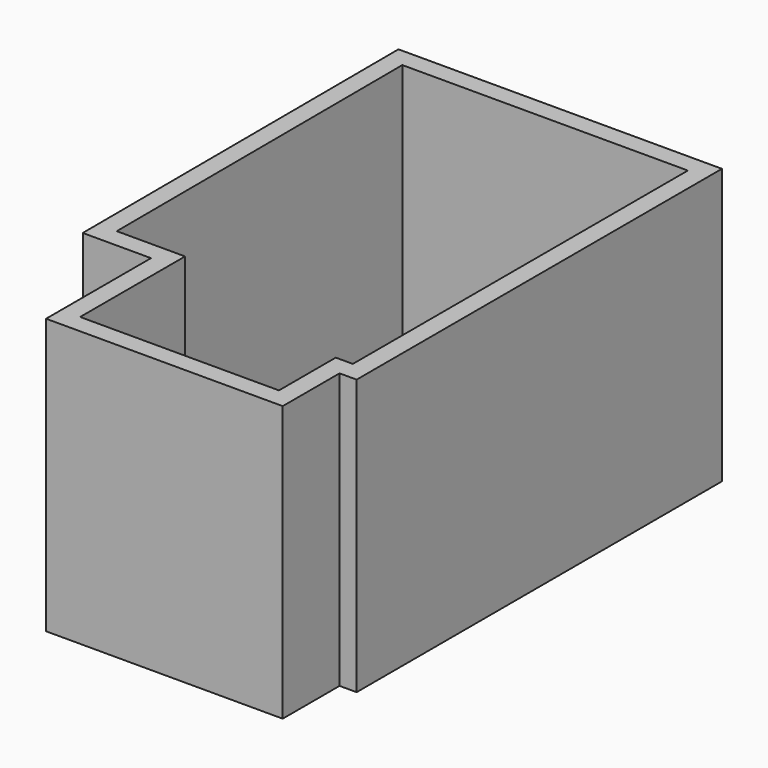
from build123d import *

# Parameters (mm, degrees)
F1_DEPTH = 25
F2_DEPTH = 2800
F3_W     = 800
F3_H     = 2000
F4_DEPTH = 199.3887424469
F5_DEPTH = 100


with BuildPart() as f1:
    # F0 (on Top) → F1 (new body)
    with BuildSketch(Plane.XY):
        Polygon((-1491.7285442352, 67.914776504), (-1477.3293733597, -3711.8628025055), (-757.3717832565, -3711.8628025055), (-757.3717832565, -5094.1815376282), (1337.7048969269, -5094.1815376282), (1337.7048969269, -4345.4256057739), (1517.6943540573, -4345.4256057739), (1517.6943540573, 67.914776504), align=None)
    extrude(amount=-F1_DEPTH)


with BuildPart() as f2:
    # F0 (on Top) → F2 (new body)
    with BuildSketch(Plane.XY):
        Polygon((1537.0936393738, -5293.5702800751), (1537.0936393738, -4544.8143482208), (1717.0830965042, -4544.8143482208), (1717.0830965042, 267.3035189509), (-1691.8783106137, 267.3035189509), (-1675.9599854953, -3911.2515449524), (-956.7605257034, -3911.2515449524), (-956.7605257034, -5293.5702800751), align=None)
        Polygon((-757.3717832565, -3711.8628025055), (-1477.3293733597, -3711.8628025055), (-1491.7285442352, 67.914776504), (1517.6943540573, 67.914776504), (1517.6943540573, -4345.4256057739), (1337.7048969269, -4345.4256057739), (1337.7048969269, -5094.1815376282), (-757.3717832565, -5094.1815376282), align=None, mode=Mode.SUBTRACT)
    extrude(amount=F2_DEPTH)

    # F3 (on face) → F4 (cut, through all)
    with BuildSketch(Plane(origin=(-956.7605257034, 0, 0), x_dir=(0, -1, 0), z_dir=(-1, 0, 0))):
        with Locations((4505.5209159851, 1000)):
            Rectangle(F3_W, F3_H)
    extrude(amount=-F4_DEPTH, mode=Mode.SUBTRACT)

    # F0 (on Top) → F5 (join)
    with BuildSketch(Plane.XY):
        Polygon((1537.0936393738, -5293.5702800751), (1537.0936393738, -4544.8143482208), (1717.0830965042, -4544.8143482208), (1717.0830965042, 267.3035189509), (-1691.8783106137, 267.3035189509), (-1675.9599854953, -3911.2515449524), (-956.7605257034, -3911.2515449524), (-956.7605257034, -5293.5702800751), align=None)
        Polygon((-757.3717832565, -3711.8628025055), (-1477.3293733597, -3711.8628025055), (-1491.7285442352, 67.914776504), (1517.6943540573, 67.914776504), (1517.6943540573, -4345.4256057739), (1337.7048969269, -4345.4256057739), (1337.7048969269, -5094.1815376282), (-757.3717832565, -5094.1815376282), align=None, mode=Mode.SUBTRACT)
        Polygon((-1491.7285442352, 67.914776504), (-1477.3293733597, -3711.8628025055), (-757.3717832565, -3711.8628025055), (-757.3717832565, -5094.1815376282), (1337.7048969269, -5094.1815376282), (1337.7048969269, -4345.4256057739), (1517.6943540573, -4345.4256057739), (1517.6943540573, 67.914776504), align=None)
    extrude(amount=-F5_DEPTH)


solid = Compound([f1.part, f2.part])
